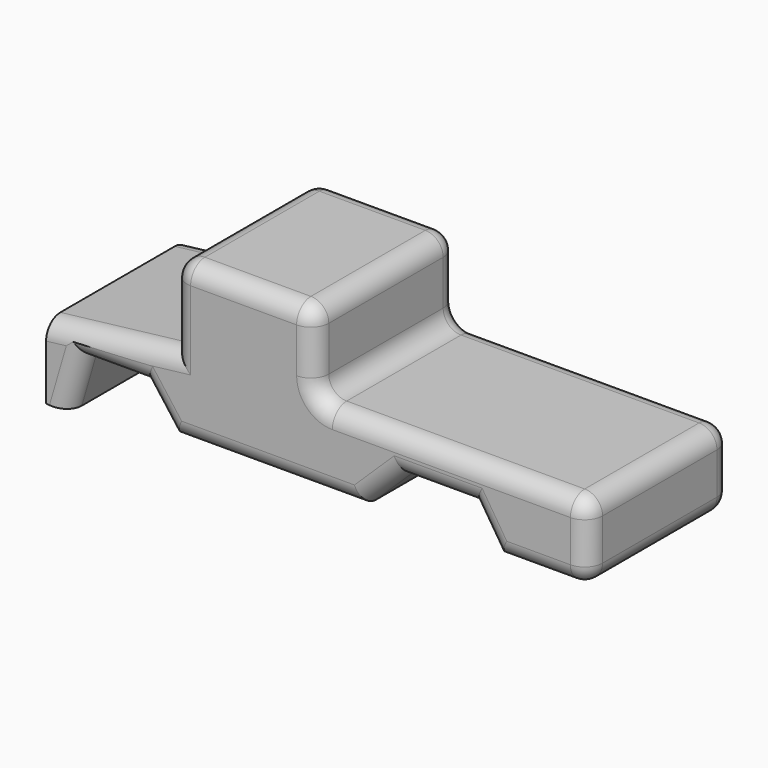
from build123d import *

# Parameters (mm, degrees)
F1_DEPTH      = 50.8
F2_T1_DEPTH   = 50.8
F2_T3_DEPTH   = 40.64
F2_T5_DEPTH   = 76.2
F2_T7_DEPTH   = 29.5973137942
F2_T9_DEPTH   = 33.5654399347
F2_T11_DEPTH  = 79.1223219872
F2_T13_DEPTH  = 47.9117414904
F2_S17_W      = 5.08
F2_S17_H      = 5.08
F2_T18_DEPTH  = 5.08
F2_S23_W      = 5.08
F2_S23_H      = 5.08
F2_T24_DEPTH  = 5.08
F2_S29_W      = 5.08
F2_S29_H      = 5.08
F2_T30_DEPTH  = 5.08
F2_S35_W      = 5.08
F2_S35_H      = 5.08
F2_T36_DEPTH  = 5.08
F2_T42_DEPTH  = 30.5130339217
F2_T47_DEPTH  = 61.6709979823
F2_T52_DEPTH  = 61.6709979823
F2_T57_DEPTH  = 30.5130339217
F2_T62_DEPTH  = 38.4398769005
F2_T67_DEPTH  = 45.5458726078
F2_T73_DEPTH  = 41.1576238629
F2_T78_DEPTH  = 38.4398769005
F2_T83_DEPTH  = 45.5458726078
F2_T89_DEPTH  = 41.1576238629
F2_T94_DEPTH  = 39.1358233333
F2_T99_DEPTH  = 42.7987075686
F2_T105_DEPTH = 40.6620223165
F2_T110_DEPTH = 39.1358233333
F2_T115_DEPTH = 42.7987075686
F2_T121_DEPTH = 40.6620223165
F2_T127_DEPTH = 30.5130339217
F2_T131_DEPTH = 61.6709979823
F2_T138_DEPTH = 30.5130339217
F2_T142_DEPTH = 61.6709979823
F2_T149_DEPTH = 38.4398769005
F2_T153_DEPTH = 45.5458726078
F2_T160_DEPTH = 41.1576238629
F2_T164_DEPTH = 45.5458726078
F2_T171_DEPTH = 38.4398769005
F2_T175_DEPTH = 45.5458726078
F2_T182_DEPTH = 41.1576238629
F2_T186_DEPTH = 45.5458726078
F2_T193_DEPTH = 42.7987075686
F2_T197_DEPTH = 39.1358233333
F2_T204_DEPTH = 40.6620223165
F2_T208_DEPTH = 42.7987075686
F2_T215_DEPTH = 42.7987075686
F2_T219_DEPTH = 39.1358233333
F2_T226_DEPTH = 40.6620223165
F2_T230_DEPTH = 42.7987075686
F2_T233_DEPTH = 12.7330339217
F2_T235_DEPTH = 67.6763198042
F2_S239_W     = 5.08
F2_S239_H     = 5.08
F2_T240_DEPTH = 5.08
F2_S245_W     = 5.08
F2_S245_H     = 5.08
F2_T246_DEPTH = 5.08
F2_S251_W     = 5.08
F2_S251_H     = 5.08
F2_T252_DEPTH = 5.08
F2_S257_W     = 5.08
F2_S257_H     = 5.08
F2_T258_DEPTH = 5.08
F2_T262_ANGLE = 90
F2_T264_ANGLE = 90


# Not quite as in the source:
# - a fillet or chamfer that OpenCascade refuses, or shapes differently, is made with other operations: its cross-section is extruded or revolved along the edge and cut away or added


with BuildPart() as f1:
    # F0 (on Front) → F1 (new body)
    with BuildSketch(Plane.XZ):
        Polygon((-106.1203256249, 11.31004747), (-106.1203256249, -9.4463042915), (-100.0155135989, -10.0567853078), (-95.7421511412, 4.5947572216), (-78.3434435725, 4.5947572216), (-70.1019465923, -6.3938992098), (-16.3796246052, -6.3938992098), (-5.0857262686, 4.5947572216), (15.0601463392, 4.5947572216), (22.0806747675, -6.3938992098), (48.0261147022, -6.3938992098), (48.0261147022, 15.5834145844), (-29.810205102, 15.5834145844), (-29.810205102, 38.4764485061), (-70.1019465923, 38.4764485061), (-70.1019465923, 15.5834145844), align=None)
    extrude(amount=F1_DEPTH)

    # F2: fillet of radius 5.08 on 33 edges, made by hand

    # F2_s2 → F2_t1 (join)
    with BuildSketch(Plane.XZ):
        with BuildLine():
            ThreePointArc((-24.730205102, 15.5834145844), (-28.3223075504, 17.071312136), (-29.810205102, 20.6634145844))
            Line((-29.810205102, 20.6634145844), (-29.810205102, 15.5834145844))
            Line((-29.810205102, 15.5834145844), (-24.730205102, 15.5834145844))
        make_face()
    extrude(amount=F2_T1_DEPTH)

    # F2_s4 → F2_t3 (cut)
    with BuildSketch(Plane.XZ.offset(5.08)):
        with BuildLine():
            ThreePointArc((-65.0219465923, 38.4764485061), (-68.6140490408, 36.9885509545), (-70.1019465923, 33.3964485061))
            Line((-70.1019465923, 33.3964485061), (-70.1019465923, 38.4764485061))
            Line((-70.1019465923, 38.4764485061), (-65.0219465923, 38.4764485061))
        make_face()
        with BuildLine():
            ThreePointArc((42.9461147022, -6.3938992098), (46.5382171507, -4.9060016582), (48.0261147022, -1.3138992098))
            Line((48.0261147022, -1.3138992098), (48.0261147022, -6.3938992098))
            Line((48.0261147022, -6.3938992098), (42.9461147022, -6.3938992098))
        make_face()
    extrude(amount=F2_T3_DEPTH, mode=Mode.SUBTRACT)

    # F2_s6 → F2_t5 (cut)
    with BuildSketch(Plane.XZ.offset(-12.7)):
        with BuildLine():
            ThreePointArc((-29.810205102, 33.3964485061), (-31.2981026535, 36.9885509545), (-34.890205102, 38.4764485061))
            Line((-34.890205102, 38.4764485061), (-29.810205102, 38.4764485061))
            Line((-29.810205102, 38.4764485061), (-29.810205102, 33.3964485061))
        make_face()
        with BuildLine():
            ThreePointArc((48.0261147022, 10.5034145844), (46.5382171507, 14.0955170328), (42.9461147022, 15.5834145844))
            Line((42.9461147022, 15.5834145844), (48.0261147022, 15.5834145844))
            Line((48.0261147022, 15.5834145844), (48.0261147022, 10.5034145844))
        make_face()
    extrude(amount=F2_T5_DEPTH, mode=Mode.SUBTRACT)

    # F2_s8 → F2_t7 (cut)
    with BuildSketch(Plane.XY.offset(-1.3138992098)):
        with BuildLine():
            ThreePointArc((48.0261147022, -5.08), (46.5382171507, -1.4878975516), (42.9461147022, 0))
            Line((42.9461147022, 0), (48.0261147022, 0))
            Line((48.0261147022, 0), (48.0261147022, -5.08))
        make_face()
        with BuildLine():
            ThreePointArc((48.0261147022, -45.72), (46.5382171507, -49.3121024484), (42.9461147022, -50.8))
            Line((42.9461147022, -50.8), (48.0261147022, -50.8))
            Line((48.0261147022, -50.8), (48.0261147022, -45.72))
        make_face()
    extrude(amount=F2_T7_DEPTH, mode=Mode.SUBTRACT)

    # F2_s10 → F2_t9 (cut)
    with BuildSketch(Plane.YZ.offset(9.3806747675)):
        with BuildLine():
            ThreePointArc((-45.72, -6.3938992098), (-49.3121024484, -4.9060016582), (-50.8, -1.3138992098))
            Line((-50.8, -1.3138992098), (-50.8, -6.3938992098))
            Line((-50.8, -6.3938992098), (-45.72, -6.3938992098))
        make_face()
        with BuildLine():
            ThreePointArc((-5.08, -6.3938992098), (-1.4878975516, -4.9060016582), (0, -1.3138992098))
            Line((0, -1.3138992098), (0, -6.3938992098))
            Line((0, -6.3938992098), (-5.08, -6.3938992098))
        make_face()
    extrude(amount=F2_T9_DEPTH, mode=Mode.SUBTRACT)

    # F2_s12 → F2_t11 (cut)
    with BuildSketch(Plane.YZ.offset(-82.8019465923)):
        with BuildLine():
            ThreePointArc((-50.8, -1.3138992098), (-49.3121024484, -4.9060016582), (-45.72, -6.3938992098))
            Line((-45.72, -6.3938992098), (-50.8, -6.3938992098))
            Line((-50.8, -6.3938992098), (-50.8, -1.3138992098))
        make_face()
        with BuildLine():
            ThreePointArc((0, -1.3138992098), (-1.4878975516, -4.9060016582), (-5.08, -6.3938992098))
            Line((-5.08, -6.3938992098), (0, -6.3938992098))
            Line((0, -6.3938992098), (0, -1.3138992098))
        make_face()
    extrude(amount=F2_T11_DEPTH, mode=Mode.SUBTRACT)

    # F2_s14 → F2_t13 (cut)
    with BuildSketch(Plane.YZ.offset(-65.0219465923)):
        with BuildLine():
            ThreePointArc((0, 33.3964485061), (-1.4878975516, 36.9885509545), (-5.08, 38.4764485061))
            Line((-5.08, 38.4764485061), (0, 38.4764485061))
            Line((0, 38.4764485061), (0, 33.3964485061))
        make_face()
        with BuildLine():
            ThreePointArc((-50.8, 33.3964485061), (-49.3121024484, 36.9885509545), (-45.72, 38.4764485061))
            Line((-45.72, 38.4764485061), (-50.8, 38.4764485061))
            Line((-50.8, 38.4764485061), (-50.8, 33.3964485061))
        make_face()
    extrude(amount=F2_T13_DEPTH, mode=Mode.SUBTRACT)


with BuildPart() as f2_tool16:
    # F2_s17 → F2_t18 (new body)
    with BuildSketch(Plane.XY.offset(33.3964485061)):
        with Locations((-67.5619465923, -2.54)):
            Rectangle(F2_S17_W, F2_S17_H)
    extrude(amount=F2_T18_DEPTH)

    # F2_s19 → F2_t20 (revolve, cut)
    with BuildSketch(Plane(origin=(-65.0219465923, -5.08, 33.3964485061), x_dir=(0.7071067812, -0.7071067812, 0), z_dir=(-0.7071067812, -0.7071067812, 0))):
        with BuildLine():
            ThreePointArc((0, -5.08), (5.08, 0), (0, 5.08))
            Line((0, 5.08), (0, -5.08))
        make_face()
    revolve(axis=Axis((-65.0219465923, -5.08, 33.3964485061), (0, 0, 1)), mode=Mode.SUBTRACT)


with BuildPart() as f1_1:
    add(f1.part)

    # F2_t15: cut F2_tool16
    add(f2_tool16.part, mode=Mode.SUBTRACT)


with BuildPart() as f2_tool22:
    # F2_s23 → F2_t24 (new body)
    with BuildSketch(Plane.XY.offset(33.3964485061)):
        with Locations((-67.5619465923, -48.26)):
            Rectangle(F2_S23_W, F2_S23_H)
    extrude(amount=F2_T24_DEPTH)

    # F2_s25 → F2_t26 (revolve, cut)
    with BuildSketch(Plane(origin=(-65.0219465923, -45.72, 33.3964485061), x_dir=(0.7071067812, 0.7071067812, 0), z_dir=(0.7071067812, -0.7071067812, 0))):
        with BuildLine():
            ThreePointArc((0, -5.08), (5.08, 0), (0, 5.08))
            Line((0, 5.08), (0, -5.08))
        make_face()
    revolve(axis=Axis((-65.0219465923, -45.72, 33.3964485061), (0, 0, 1)), mode=Mode.SUBTRACT)


with BuildPart() as f1_2:
    add(f1_1.part)

    # F2_t21: cut F2_tool22
    add(f2_tool22.part, mode=Mode.SUBTRACT)


with BuildPart() as f2_tool28:
    # F2_s29 → F2_t30 (new body)
    with BuildSketch(Plane.XY.offset(-1.3138992098)):
        with Locations((45.4861147022, -2.54)):
            Rectangle(F2_S29_W, F2_S29_H)
    extrude(amount=-F2_T30_DEPTH)

    # F2_s31 → F2_t32 (revolve, cut)
    with BuildSketch(Plane(origin=(42.9461147022, -5.08, -1.3138992098), x_dir=(-0.7071067812, -0.7071067812, 0), z_dir=(0.7071067812, -0.7071067812, 0))):
        with BuildLine():
            ThreePointArc((0, -5.08), (5.08, 0), (0, 5.08))
            Line((0, 5.08), (0, -5.08))
        make_face()
    revolve(axis=Axis((42.9461147022, -5.08, -1.3138992098), (0, 0, -1)), mode=Mode.SUBTRACT)


with BuildPart() as f1_3:
    add(f1_2.part)

    # F2_t27: cut F2_tool28
    add(f2_tool28.part, mode=Mode.SUBTRACT)


with BuildPart() as f2_tool34:
    # F2_s35 → F2_t36 (new body)
    with BuildSketch(Plane.XY.offset(-1.3138992098)):
        with Locations((45.4861147022, -48.26)):
            Rectangle(F2_S35_W, F2_S35_H)
    extrude(amount=-F2_T36_DEPTH)

    # F2_s37 → F2_t38 (revolve, cut)
    with BuildSketch(Plane(origin=(42.9461147022, -45.72, -1.3138992098), x_dir=(-0.7071067812, 0.7071067812, 0), z_dir=(-0.7071067812, -0.7071067812, 0))):
        with BuildLine():
            ThreePointArc((0, -5.08), (5.08, 0), (0, 5.08))
            Line((0, 5.08), (0, -5.08))
        make_face()
    revolve(axis=Axis((42.9461147022, -45.72, -1.3138992098), (0, 0, -1)), mode=Mode.SUBTRACT)


with BuildPart() as f1_4:
    add(f1_3.part)

    # F2_t33: cut F2_tool34
    add(f2_tool34.part, mode=Mode.SUBTRACT)


with BuildPart() as f2_tool40:
    # F2_s41 → F2_t42 (new body)
    with BuildSketch(Plane.XY.offset(33.3964485061)):
        with BuildLine():
            ThreePointArc((-65.0219465923, 0), (-68.6140490408, -1.4878975516), (-70.1019465923, -5.08))
            Line((-70.1019465923, -5.08), (-70.1019465923, 0))
            Line((-70.1019465923, 0), (-65.0219465923, 0))
        make_face()
    extrude(amount=-F2_T42_DEPTH)

    split(bisect_by=Plane(origin=(-2.796301967, 0, 23.5688302549), x_dir=(0, 1, 0), z_dir=(-0.1178177429, 0, 0.9930352358)), keep=Keep.TOP)


with BuildPart() as f1_5:
    add(f1_4.part)

    # F2_t39: cut F2_tool40
    add(f2_tool40.part, mode=Mode.SUBTRACT)


with BuildPart() as f2_tool45:
    # F2_s46 → F2_t47 (new body)
    with BuildSketch(Plane(origin=(-54.6940971312, 0, -6.4891303359), x_dir=(0, 1, 0), z_dir=(-0.9930352358, 0, -0.1178177429))):
        with BuildLine():
            ThreePointArc((0, -18.6541328949), (-1.4878975516, -22.2462353434), (-5.08, -23.7341328949))
            Line((-5.08, -23.7341328949), (0, -23.7341328949))
            Line((0, -23.7341328949), (0, -18.6541328949))
        make_face()
    extrude(amount=F2_T47_DEPTH)

    split(bisect_by=Plane.YZ.offset(-70.1019465923), keep=Keep.BOTTOM)


with BuildPart() as f1_6:
    add(f1_5.part)

    # F2_t44: cut F2_tool45
    add(f2_tool45.part, mode=Mode.SUBTRACT)


with BuildPart() as f2_tool50:
    # F2_s51 → F2_t52 (new body)
    with BuildSketch(Plane(origin=(-54.6940971312, 0, -6.4891303359), x_dir=(0, 1, 0), z_dir=(-0.9930352358, 0, -0.1178177429))):
        with BuildLine():
            ThreePointArc((-50.8, -18.6541328949), (-49.3121024484, -22.2462353434), (-45.72, -23.7341328949))
            Line((-45.72, -23.7341328949), (-50.8, -23.7341328949))
            Line((-50.8, -23.7341328949), (-50.8, -18.6541328949))
        make_face()
    extrude(amount=F2_T52_DEPTH)

    split(bisect_by=Plane.YZ.offset(-70.1019465923), keep=Keep.BOTTOM)


with BuildPart() as f1_7:
    add(f1_6.part)

    # F2_t49: cut F2_tool50
    add(f2_tool50.part, mode=Mode.SUBTRACT)


with BuildPart() as f2_tool55:
    # F2_s56 → F2_t57 (new body)
    with BuildSketch(Plane.XY.offset(33.3964485061)):
        with BuildLine():
            ThreePointArc((-65.0219465923, -50.8), (-68.6140490408, -49.3121024484), (-70.1019465923, -45.72))
            Line((-70.1019465923, -45.72), (-70.1019465923, -50.8))
            Line((-70.1019465923, -50.8), (-65.0219465923, -50.8))
        make_face()
    extrude(amount=-F2_T57_DEPTH)

    split(bisect_by=Plane(origin=(-2.796301967, 0, 23.5688302549), x_dir=(0, 1, 0), z_dir=(-0.1178177429, 0, 0.9930352358)), keep=Keep.TOP)


with BuildPart() as f1_8:
    add(f1_7.part)

    # F2_t54: cut F2_tool55
    add(f2_tool55.part, mode=Mode.SUBTRACT)


with BuildPart() as f2_tool60:
    # F2_s61 → F2_t62 (new body)
    with BuildSketch(Plane(origin=(-4.5567996099, 0, 7.1323841007), x_dir=(0, 1, 0), z_dir=(0.5383891644, 0, -0.8426963318))):
        with BuildLine():
            ThreePointArc((-45.72, 15.1648975779), (-49.3121024484, 16.6527951295), (-50.8, 20.2448975779))
            Line((-50.8, 20.2448975779), (-50.8, 15.1648975779))
            Line((-50.8, 15.1648975779), (-45.72, 15.1648975779))
        make_face()
    extrude(amount=F2_T62_DEPTH)

    split(bisect_by=Plane.XY.offset(4.5947572216), keep=Keep.BOTTOM)


with BuildPart() as f1_9:
    add(f1_8.part)

    # F2_t59: cut F2_tool60
    add(f2_tool60.part, mode=Mode.SUBTRACT)


with BuildPart() as f2_tool65:
    # F2_s66 → F2_t67 (new body)
    with BuildSketch(Plane.YZ.offset(-17.7857262686)):
        with BuildLine():
            ThreePointArc((-50.8, 9.6747572216), (-49.3121024484, 6.0826547732), (-45.72, 4.5947572216))
            Line((-45.72, 4.5947572216), (-50.8, 4.5947572216))
            Line((-50.8, 4.5947572216), (-50.8, 9.6747572216))
        make_face()
    extrude(amount=F2_T67_DEPTH)

    split(bisect_by=Plane(origin=(12.7794035613, 0, 8.1646165351), x_dir=(0, 1, 0), z_dir=(-0.8426963318, 0, -0.5383891644)), keep=Keep.TOP)

    split(bisect_by=Plane(origin=(-4.769724943, 0, 4.9022179314), x_dir=(0, 1, 0), z_dir=(0.6973549139, 0, -0.7167259756)), keep=Keep.TOP)


with BuildPart() as f1_10:
    add(f1_9.part)

    # F2_t64: cut F2_tool65
    add(f2_tool65.part, mode=Mode.SUBTRACT)


with BuildPart() as f2_tool71:
    # F2_s72 → F2_t73 (new body)
    with BuildSketch(Plane(origin=(-20.7123195525, 0, -20.1525245471), x_dir=(0, 1, 0), z_dir=(0.7167259756, 0, 0.6973549139))):
        with BuildLine():
            ThreePointArc((-50.8, 11.9197380563), (-49.3121024484, 8.3276356079), (-45.72, 6.8397380563))
            Line((-45.72, 6.8397380563), (-50.8, 6.8397380563))
            Line((-50.8, 6.8397380563), (-50.8, 11.9197380563))
        make_face()
    extrude(amount=F2_T73_DEPTH)

    split(bisect_by=Plane.XY.offset(4.5947572216), keep=Keep.BOTTOM)


with BuildPart() as f1_11:
    add(f1_10.part)

    # F2_t70: cut F2_tool71
    add(f2_tool71.part, mode=Mode.SUBTRACT)


with BuildPart() as f2_tool76:
    # F2_s77 → F2_t78 (new body)
    with BuildSketch(Plane(origin=(-4.5567996099, 0, 7.1323841007), x_dir=(0, 1, 0), z_dir=(0.5383891644, 0, -0.8426963318))):
        with BuildLine():
            ThreePointArc((-5.08, 15.1648975779), (-1.4878975516, 16.6527951295), (0, 20.2448975779))
            Line((0, 20.2448975779), (0, 15.1648975779))
            Line((0, 15.1648975779), (-5.08, 15.1648975779))
        make_face()
    extrude(amount=F2_T78_DEPTH)

    split(bisect_by=Plane.XY.offset(4.5947572216), keep=Keep.BOTTOM)


with BuildPart() as f1_12:
    add(f1_11.part)

    # F2_t75: cut F2_tool76
    add(f2_tool76.part, mode=Mode.SUBTRACT)


with BuildPart() as f2_tool81:
    # F2_s82 → F2_t83 (new body)
    with BuildSketch(Plane.YZ.offset(-17.7857262686)):
        with BuildLine():
            ThreePointArc((0, 9.6747572216), (-1.4878975516, 6.0826547732), (-5.08, 4.5947572216))
            Line((-5.08, 4.5947572216), (0, 4.5947572216))
            Line((0, 4.5947572216), (0, 9.6747572216))
        make_face()
    extrude(amount=F2_T83_DEPTH)

    split(bisect_by=Plane(origin=(12.7794035613, 0, 8.1646165351), x_dir=(0, 1, 0), z_dir=(-0.8426963318, 0, -0.5383891644)), keep=Keep.TOP)

    split(bisect_by=Plane(origin=(-4.769724943, 0, 4.9022179314), x_dir=(0, 1, 0), z_dir=(0.6973549139, 0, -0.7167259756)), keep=Keep.TOP)


with BuildPart() as f1_13:
    add(f1_12.part)

    # F2_t80: cut F2_tool81
    add(f2_tool81.part, mode=Mode.SUBTRACT)


with BuildPart() as f2_tool87:
    # F2_s88 → F2_t89 (new body)
    with BuildSketch(Plane(origin=(-20.7123195525, 0, -20.1525245471), x_dir=(0, 1, 0), z_dir=(0.7167259756, 0, 0.6973549139))):
        with BuildLine():
            ThreePointArc((0, 11.9197380563), (-1.4878975516, 8.3276356079), (-5.08, 6.8397380563))
            Line((-5.08, 6.8397380563), (0, 6.8397380563))
            Line((0, 6.8397380563), (0, 11.9197380563))
        make_face()
    extrude(amount=F2_T89_DEPTH)

    split(bisect_by=Plane.XY.offset(4.5947572216), keep=Keep.BOTTOM)


with BuildPart() as f1_14:
    add(f1_13.part)

    # F2_t86: cut F2_tool87
    add(f2_tool87.part, mode=Mode.SUBTRACT)


with BuildPart() as f2_tool92:
    # F2_s93 → F2_t94 (new body)
    with BuildSketch(Plane(origin=(-38.0291466545, 0, 50.705500223), x_dir=(0, 1, 0), z_dir=(0.600000217, 0, -0.7999998373))):
        with BuildLine():
            ThreePointArc((-50.8, -54.8378867796), (-49.3121024484, -58.429989228), (-45.72, -59.9178867796))
            Line((-45.72, -59.9178867796), (-50.8, -59.9178867796))
            Line((-50.8, -59.9178867796), (-50.8, -54.8378867796))
        make_face()
    extrude(amount=F2_T94_DEPTH)

    split(bisect_by=Plane.XY.offset(4.5947572216), keep=Keep.BOTTOM)


with BuildPart() as f1_15:
    add(f1_14.part)

    # F2_t91: cut F2_tool92
    add(f2_tool92.part, mode=Mode.SUBTRACT)


with BuildPart() as f2_tool97:
    # F2_s98 → F2_t99 (new body)
    with BuildSketch(Plane.YZ.offset(-108.4421511412)):
        with BuildLine():
            ThreePointArc((-50.8, 9.6747572216), (-49.3121024484, 6.0826547732), (-45.72, 4.5947572216))
            Line((-45.72, 4.5947572216), (-50.8, 4.5947572216))
            Line((-50.8, 4.5947572216), (-50.8, 9.6747572216))
        make_face()
    extrude(amount=F2_T99_DEPTH)

    split(bisect_by=Plane(origin=(-89.4710495478, 0, 26.0956976663), x_dir=(0, 1, 0), z_dir=(0.9600000724, 0, -0.2799997516)), keep=Keep.TOP)

    split(bisect_by=Plane(origin=(-47.9342996735, 0, -35.950745068), x_dir=(0, 1, 0), z_dir=(-0.7999998373, 0, -0.600000217)), keep=Keep.TOP)


with BuildPart() as f1_16:
    add(f1_15.part)

    # F2_t96: cut F2_tool97
    add(f2_tool97.part, mode=Mode.SUBTRACT)


with BuildPart() as f2_tool103:
    # F2_s104 → F2_t105 (new body)
    with BuildSketch(Plane(origin=(-14.1004608967, 0, -48.3444838941), x_dir=(0, 1, 0), z_dir=(0.2799997516, 0, 0.9600000724))):
        with BuildLine():
            ThreePointArc((-50.8, 98.2790029124), (-49.3121024484, 94.686900464), (-45.72, 93.1990029124))
            Line((-45.72, 93.1990029124), (-50.8, 93.1990029124))
            Line((-50.8, 93.1990029124), (-50.8, 98.2790029124))
        make_face()
    extrude(amount=F2_T105_DEPTH)

    split(bisect_by=Plane.XY.offset(4.5947572216), keep=Keep.BOTTOM)


with BuildPart() as f1_17:
    add(f1_16.part)

    # F2_t102: cut F2_tool103
    add(f2_tool103.part, mode=Mode.SUBTRACT)


with BuildPart() as f2_tool108:
    # F2_s109 → F2_t110 (new body)
    with BuildSketch(Plane(origin=(-38.0291466545, 0, 50.705500223), x_dir=(0, 1, 0), z_dir=(0.600000217, 0, -0.7999998373))):
        with BuildLine():
            ThreePointArc((0, -54.8378867796), (-1.4878975516, -58.429989228), (-5.08, -59.9178867796))
            Line((-5.08, -59.9178867796), (0, -59.9178867796))
            Line((0, -59.9178867796), (0, -54.8378867796))
        make_face()
    extrude(amount=F2_T110_DEPTH)

    split(bisect_by=Plane.XY.offset(4.5947572216), keep=Keep.BOTTOM)


with BuildPart() as f1_18:
    add(f1_17.part)

    # F2_t107: cut F2_tool108
    add(f2_tool108.part, mode=Mode.SUBTRACT)


with BuildPart() as f2_tool113:
    # F2_s114 → F2_t115 (new body)
    with BuildSketch(Plane.YZ.offset(-108.4421511412)):
        with BuildLine():
            ThreePointArc((0, 9.6747572216), (-1.4878975516, 6.0826547732), (-5.08, 4.5947572216))
            Line((-5.08, 4.5947572216), (0, 4.5947572216))
            Line((0, 4.5947572216), (0, 9.6747572216))
        make_face()
    extrude(amount=F2_T115_DEPTH)

    split(bisect_by=Plane(origin=(-89.4710495478, 0, 26.0956976663), x_dir=(0, 1, 0), z_dir=(0.9600000724, 0, -0.2799997516)), keep=Keep.TOP)

    split(bisect_by=Plane(origin=(-47.9342996735, 0, -35.950745068), x_dir=(0, 1, 0), z_dir=(-0.7999998373, 0, -0.600000217)), keep=Keep.TOP)


with BuildPart() as f1_19:
    add(f1_18.part)

    # F2_t112: cut F2_tool113
    add(f2_tool113.part, mode=Mode.SUBTRACT)


with BuildPart() as f2_tool119:
    # F2_s120 → F2_t121 (new body)
    with BuildSketch(Plane(origin=(-14.1004608967, 0, -48.3444838941), x_dir=(0, 1, 0), z_dir=(0.2799997516, 0, 0.9600000724))):
        with BuildLine():
            ThreePointArc((0, 98.2790029124), (-1.4878975516, 94.686900464), (-5.08, 93.1990029124))
            Line((-5.08, 93.1990029124), (0, 93.1990029124))
            Line((0, 93.1990029124), (0, 98.2790029124))
        make_face()
    extrude(amount=F2_T121_DEPTH)

    split(bisect_by=Plane.XY.offset(4.5947572216), keep=Keep.BOTTOM)


with BuildPart() as f1_20:
    add(f1_19.part)

    # F2_t118: cut F2_tool119
    add(f2_tool119.part, mode=Mode.SUBTRACT)


with BuildPart() as f2_tool125:
    # F2_s126 → F2_t127 (new body)
    with BuildSketch(Plane.XY.offset(33.3964485061)):
        with BuildLine():
            ThreePointArc((-65.0219465923, 0), (-68.6140490408, -1.4878975516), (-70.1019465923, -5.08))
            Line((-70.1019465923, -5.08), (-70.1019465923, 0))
            Line((-70.1019465923, 0), (-65.0219465923, 0))
        make_face()
    extrude(amount=-F2_T127_DEPTH)

    split(bisect_by=Plane(origin=(-2.796301967, 0, 23.5688302549), x_dir=(0, 1, 0), z_dir=(0.1178177429, 0, -0.9930352358)), keep=Keep.TOP)


with BuildPart() as f2_tool129:
    # F2_s130 → F2_t131 (new body)
    with BuildSketch(Plane(origin=(-54.6940971312, 0, -6.4891303359), x_dir=(0, 1, 0), z_dir=(-0.9930352358, 0, -0.1178177429))):
        with BuildLine():
            ThreePointArc((0, -18.6541328949), (-1.4878975516, -22.2462353434), (-5.08, -23.7341328949))
            Line((-5.08, -23.7341328949), (0, -23.7341328949))
            Line((0, -23.7341328949), (0, -18.6541328949))
        make_face()
    extrude(amount=F2_T131_DEPTH)

    split(bisect_by=Plane.YZ.offset(-70.1019465923), keep=Keep.TOP)


with BuildPart() as f2_tool125_1:
    add(f2_tool125.part)

    # F2_t133: intersect F2_tool129
    add(f2_tool129.part, mode=Mode.INTERSECT)


with BuildPart() as f1_21:
    add(f1_20.part)

    # F2_t123: cut F2_tool125
    add(f2_tool125_1.part, mode=Mode.SUBTRACT)


with BuildPart() as f2_tool136:
    # F2_s137 → F2_t138 (new body)
    with BuildSketch(Plane.XY.offset(33.3964485061)):
        with BuildLine():
            ThreePointArc((-65.0219465923, -50.8), (-68.6140490408, -49.3121024484), (-70.1019465923, -45.72))
            Line((-70.1019465923, -45.72), (-70.1019465923, -50.8))
            Line((-70.1019465923, -50.8), (-65.0219465923, -50.8))
        make_face()
    extrude(amount=-F2_T138_DEPTH)

    split(bisect_by=Plane(origin=(-2.796301967, 0, 23.5688302549), x_dir=(0, 1, 0), z_dir=(0.1178177429, 0, -0.9930352358)), keep=Keep.TOP)


with BuildPart() as f2_tool140:
    # F2_s141 → F2_t142 (new body)
    with BuildSketch(Plane(origin=(-54.6940971312, 0, -6.4891303359), x_dir=(0, 1, 0), z_dir=(-0.9930352358, 0, -0.1178177429))):
        with BuildLine():
            ThreePointArc((-50.8, -18.6541328949), (-49.3121024484, -22.2462353434), (-45.72, -23.7341328949))
            Line((-45.72, -23.7341328949), (-50.8, -23.7341328949))
            Line((-50.8, -23.7341328949), (-50.8, -18.6541328949))
        make_face()
    extrude(amount=F2_T142_DEPTH)

    split(bisect_by=Plane.YZ.offset(-70.1019465923), keep=Keep.TOP)


with BuildPart() as f2_tool136_1:
    add(f2_tool136.part)

    # F2_t144: intersect F2_tool140
    add(f2_tool140.part, mode=Mode.INTERSECT)


with BuildPart() as f1_22:
    add(f1_21.part)

    # F2_t134: cut F2_tool136
    add(f2_tool136_1.part, mode=Mode.SUBTRACT)


with BuildPart() as f2_tool147:
    # F2_s148 → F2_t149 (new body)
    with BuildSketch(Plane(origin=(-4.5567996099, 0, 7.1323841007), x_dir=(0, 1, 0), z_dir=(0.5383891644, 0, -0.8426963318))):
        with BuildLine():
            ThreePointArc((-45.72, 15.1648975779), (-49.3121024484, 16.6527951295), (-50.8, 20.2448975779))
            Line((-50.8, 20.2448975779), (-50.8, 15.1648975779))
            Line((-50.8, 15.1648975779), (-45.72, 15.1648975779))
        make_face()
    extrude(amount=F2_T149_DEPTH)

    split(bisect_by=Plane.XY.offset(4.5947572216), keep=Keep.TOP)


with BuildPart() as f2_tool151:
    # F2_s152 → F2_t153 (new body)
    with BuildSketch(Plane.YZ.offset(-17.7857262686)):
        with BuildLine():
            ThreePointArc((-50.8, 9.6747572216), (-49.3121024484, 6.0826547732), (-45.72, 4.5947572216))
            Line((-45.72, 4.5947572216), (-50.8, 4.5947572216))
            Line((-50.8, 4.5947572216), (-50.8, 9.6747572216))
        make_face()
    extrude(amount=F2_T153_DEPTH)

    split(bisect_by=Plane(origin=(12.7794035613, 0, 8.1646165351), x_dir=(0, 1, 0), z_dir=(0.8426963318, 0, 0.5383891644)), keep=Keep.TOP)


with BuildPart() as f2_tool147_1:
    add(f2_tool147.part)

    # F2_t155: intersect F2_tool151
    add(f2_tool151.part, mode=Mode.INTERSECT)


with BuildPart() as f1_23:
    add(f1_22.part)

    # F2_t145: cut F2_tool147
    add(f2_tool147_1.part, mode=Mode.SUBTRACT)


with BuildPart() as f2_tool158:
    # F2_s159 → F2_t160 (new body)
    with BuildSketch(Plane(origin=(-20.7123195525, 0, -20.1525245471), x_dir=(0, 1, 0), z_dir=(0.7167259756, 0, 0.6973549139))):
        with BuildLine():
            ThreePointArc((-50.8, 11.9197380563), (-49.3121024484, 8.3276356079), (-45.72, 6.8397380563))
            Line((-45.72, 6.8397380563), (-50.8, 6.8397380563))
            Line((-50.8, 6.8397380563), (-50.8, 11.9197380563))
        make_face()
    extrude(amount=F2_T160_DEPTH)

    split(bisect_by=Plane.XY.offset(4.5947572216), keep=Keep.TOP)


with BuildPart() as f2_tool162:
    # F2_s163 → F2_t164 (new body)
    with BuildSketch(Plane.YZ.offset(-17.7857262686)):
        with BuildLine():
            ThreePointArc((-50.8, 9.6747572216), (-49.3121024484, 6.0826547732), (-45.72, 4.5947572216))
            Line((-45.72, 4.5947572216), (-50.8, 4.5947572216))
            Line((-50.8, 4.5947572216), (-50.8, 9.6747572216))
        make_face()
    extrude(amount=F2_T164_DEPTH)

    split(bisect_by=Plane(origin=(-4.769724943, 0, 4.9022179314), x_dir=(0, 1, 0), z_dir=(-0.6973549139, 0, 0.7167259756)), keep=Keep.TOP)


with BuildPart() as f2_tool158_1:
    add(f2_tool158.part)

    # F2_t166: intersect F2_tool162
    add(f2_tool162.part, mode=Mode.INTERSECT)


with BuildPart() as f1_24:
    add(f1_23.part)

    # F2_t156: cut F2_tool158
    add(f2_tool158_1.part, mode=Mode.SUBTRACT)


with BuildPart() as f2_tool169:
    # F2_s170 → F2_t171 (new body)
    with BuildSketch(Plane(origin=(-4.5567996099, 0, 7.1323841007), x_dir=(0, 1, 0), z_dir=(0.5383891644, 0, -0.8426963318))):
        with BuildLine():
            ThreePointArc((-5.08, 15.1648975779), (-1.4878975516, 16.6527951295), (0, 20.2448975779))
            Line((0, 20.2448975779), (0, 15.1648975779))
            Line((0, 15.1648975779), (-5.08, 15.1648975779))
        make_face()
    extrude(amount=F2_T171_DEPTH)

    split(bisect_by=Plane.XY.offset(4.5947572216), keep=Keep.TOP)


with BuildPart() as f2_tool173:
    # F2_s174 → F2_t175 (new body)
    with BuildSketch(Plane.YZ.offset(-17.7857262686)):
        with BuildLine():
            ThreePointArc((0, 9.6747572216), (-1.4878975516, 6.0826547732), (-5.08, 4.5947572216))
            Line((-5.08, 4.5947572216), (0, 4.5947572216))
            Line((0, 4.5947572216), (0, 9.6747572216))
        make_face()
    extrude(amount=F2_T175_DEPTH)

    split(bisect_by=Plane(origin=(12.7794035613, 0, 8.1646165351), x_dir=(0, 1, 0), z_dir=(0.8426963318, 0, 0.5383891644)), keep=Keep.TOP)


with BuildPart() as f2_tool169_1:
    add(f2_tool169.part)

    # F2_t177: intersect F2_tool173
    add(f2_tool173.part, mode=Mode.INTERSECT)


with BuildPart() as f1_25:
    add(f1_24.part)

    # F2_t167: cut F2_tool169
    add(f2_tool169_1.part, mode=Mode.SUBTRACT)


with BuildPart() as f2_tool180:
    # F2_s181 → F2_t182 (new body)
    with BuildSketch(Plane(origin=(-20.7123195525, 0, -20.1525245471), x_dir=(0, 1, 0), z_dir=(0.7167259756, 0, 0.6973549139))):
        with BuildLine():
            ThreePointArc((0, 11.9197380563), (-1.4878975516, 8.3276356079), (-5.08, 6.8397380563))
            Line((-5.08, 6.8397380563), (0, 6.8397380563))
            Line((0, 6.8397380563), (0, 11.9197380563))
        make_face()
    extrude(amount=F2_T182_DEPTH)

    split(bisect_by=Plane.XY.offset(4.5947572216), keep=Keep.TOP)


with BuildPart() as f2_tool184:
    # F2_s185 → F2_t186 (new body)
    with BuildSketch(Plane.YZ.offset(-17.7857262686)):
        with BuildLine():
            ThreePointArc((0, 9.6747572216), (-1.4878975516, 6.0826547732), (-5.08, 4.5947572216))
            Line((-5.08, 4.5947572216), (0, 4.5947572216))
            Line((0, 4.5947572216), (0, 9.6747572216))
        make_face()
    extrude(amount=F2_T186_DEPTH)

    split(bisect_by=Plane(origin=(-4.769724943, 0, 4.9022179314), x_dir=(0, 1, 0), z_dir=(-0.6973549139, 0, 0.7167259756)), keep=Keep.TOP)


with BuildPart() as f2_tool180_1:
    add(f2_tool180.part)

    # F2_t188: intersect F2_tool184
    add(f2_tool184.part, mode=Mode.INTERSECT)


with BuildPart() as f1_26:
    add(f1_25.part)

    # F2_t178: cut F2_tool180
    add(f2_tool180_1.part, mode=Mode.SUBTRACT)


with BuildPart() as f2_tool191:
    # F2_s192 → F2_t193 (new body)
    with BuildSketch(Plane.YZ.offset(-108.4421511412)):
        with BuildLine():
            ThreePointArc((-50.8, 9.6747572216), (-49.3121024484, 6.0826547732), (-45.72, 4.5947572216))
            Line((-45.72, 4.5947572216), (-50.8, 4.5947572216))
            Line((-50.8, 4.5947572216), (-50.8, 9.6747572216))
        make_face()
    extrude(amount=F2_T193_DEPTH)

    split(bisect_by=Plane(origin=(-47.9342996735, 0, -35.950745068), x_dir=(0, 1, 0), z_dir=(0.7999998373, 0, 0.600000217)), keep=Keep.TOP)


with BuildPart() as f2_tool195:
    # F2_s196 → F2_t197 (new body)
    with BuildSketch(Plane(origin=(-38.0291466545, 0, 50.705500223), x_dir=(0, 1, 0), z_dir=(0.600000217, 0, -0.7999998373))):
        with BuildLine():
            ThreePointArc((-50.8, -54.8378867796), (-49.3121024484, -58.429989228), (-45.72, -59.9178867796))
            Line((-45.72, -59.9178867796), (-50.8, -59.9178867796))
            Line((-50.8, -59.9178867796), (-50.8, -54.8378867796))
        make_face()
    extrude(amount=F2_T197_DEPTH)

    split(bisect_by=Plane.XY.offset(4.5947572216), keep=Keep.TOP)


with BuildPart() as f2_tool191_1:
    add(f2_tool191.part)

    # F2_t199: intersect F2_tool195
    add(f2_tool195.part, mode=Mode.INTERSECT)


with BuildPart() as f1_27:
    add(f1_26.part)

    # F2_t189: cut F2_tool191
    add(f2_tool191_1.part, mode=Mode.SUBTRACT)


with BuildPart() as f2_tool202:
    # F2_s203 → F2_t204 (new body)
    with BuildSketch(Plane(origin=(-14.1004608967, 0, -48.3444838941), x_dir=(0, 1, 0), z_dir=(0.2799997516, 0, 0.9600000724))):
        with BuildLine():
            ThreePointArc((-50.8, 98.2790029124), (-49.3121024484, 94.686900464), (-45.72, 93.1990029124))
            Line((-45.72, 93.1990029124), (-50.8, 93.1990029124))
            Line((-50.8, 93.1990029124), (-50.8, 98.2790029124))
        make_face()
    extrude(amount=F2_T204_DEPTH)

    split(bisect_by=Plane.XY.offset(4.5947572216), keep=Keep.TOP)


with BuildPart() as f2_tool206:
    # F2_s207 → F2_t208 (new body)
    with BuildSketch(Plane.YZ.offset(-108.4421511412)):
        with BuildLine():
            ThreePointArc((-50.8, 9.6747572216), (-49.3121024484, 6.0826547732), (-45.72, 4.5947572216))
            Line((-45.72, 4.5947572216), (-50.8, 4.5947572216))
            Line((-50.8, 4.5947572216), (-50.8, 9.6747572216))
        make_face()
    extrude(amount=F2_T208_DEPTH)

    split(bisect_by=Plane(origin=(-89.4710495478, 0, 26.0956976663), x_dir=(0, 1, 0), z_dir=(-0.9600000724, 0, 0.2799997516)), keep=Keep.TOP)


with BuildPart() as f2_tool202_1:
    add(f2_tool202.part)

    # F2_t210: intersect F2_tool206
    add(f2_tool206.part, mode=Mode.INTERSECT)


with BuildPart() as f1_28:
    add(f1_27.part)

    # F2_t200: cut F2_tool202
    add(f2_tool202_1.part, mode=Mode.SUBTRACT)


with BuildPart() as f2_tool213:
    # F2_s214 → F2_t215 (new body)
    with BuildSketch(Plane.YZ.offset(-108.4421511412)):
        with BuildLine():
            ThreePointArc((0, 9.6747572216), (-1.4878975516, 6.0826547732), (-5.08, 4.5947572216))
            Line((-5.08, 4.5947572216), (0, 4.5947572216))
            Line((0, 4.5947572216), (0, 9.6747572216))
        make_face()
    extrude(amount=F2_T215_DEPTH)

    split(bisect_by=Plane(origin=(-47.9342996735, 0, -35.950745068), x_dir=(0, 1, 0), z_dir=(0.7999998373, 0, 0.600000217)), keep=Keep.TOP)


with BuildPart() as f2_tool217:
    # F2_s218 → F2_t219 (new body)
    with BuildSketch(Plane(origin=(-38.0291466545, 0, 50.705500223), x_dir=(0, 1, 0), z_dir=(0.600000217, 0, -0.7999998373))):
        with BuildLine():
            ThreePointArc((0, -54.8378867796), (-1.4878975516, -58.429989228), (-5.08, -59.9178867796))
            Line((-5.08, -59.9178867796), (0, -59.9178867796))
            Line((0, -59.9178867796), (0, -54.8378867796))
        make_face()
    extrude(amount=F2_T219_DEPTH)

    split(bisect_by=Plane.XY.offset(4.5947572216), keep=Keep.TOP)


with BuildPart() as f2_tool213_1:
    add(f2_tool213.part)

    # F2_t221: intersect F2_tool217
    add(f2_tool217.part, mode=Mode.INTERSECT)


with BuildPart() as f1_29:
    add(f1_28.part)

    # F2_t211: cut F2_tool213
    add(f2_tool213_1.part, mode=Mode.SUBTRACT)


with BuildPart() as f2_tool224:
    # F2_s225 → F2_t226 (new body)
    with BuildSketch(Plane(origin=(-14.1004608967, 0, -48.3444838941), x_dir=(0, 1, 0), z_dir=(0.2799997516, 0, 0.9600000724))):
        with BuildLine():
            ThreePointArc((0, 98.2790029124), (-1.4878975516, 94.686900464), (-5.08, 93.1990029124))
            Line((-5.08, 93.1990029124), (0, 93.1990029124))
            Line((0, 93.1990029124), (0, 98.2790029124))
        make_face()
    extrude(amount=F2_T226_DEPTH)

    split(bisect_by=Plane.XY.offset(4.5947572216), keep=Keep.TOP)


with BuildPart() as f2_tool228:
    # F2_s229 → F2_t230 (new body)
    with BuildSketch(Plane.YZ.offset(-108.4421511412)):
        with BuildLine():
            ThreePointArc((0, 9.6747572216), (-1.4878975516, 6.0826547732), (-5.08, 4.5947572216))
            Line((-5.08, 4.5947572216), (0, 4.5947572216))
            Line((0, 4.5947572216), (0, 9.6747572216))
        make_face()
    extrude(amount=F2_T230_DEPTH)

    split(bisect_by=Plane(origin=(-89.4710495478, 0, 26.0956976663), x_dir=(0, 1, 0), z_dir=(-0.9600000724, 0, 0.2799997516)), keep=Keep.TOP)


with BuildPart() as f2_tool224_1:
    add(f2_tool224.part)

    # F2_t232: intersect F2_tool228
    add(f2_tool228.part, mode=Mode.INTERSECT)


with BuildPart() as f1_30:
    add(f1_29.part)

    # F2_t222: cut F2_tool224
    add(f2_tool224_1.part, mode=Mode.SUBTRACT)

    # F2_s234 → F2_t233 (cut)
    with BuildSketch(Plane.XY.offset(20.6634145844)):
        with BuildLine():
            ThreePointArc((-34.890205102, -50.8), (-31.2981026535, -49.3121024484), (-29.810205102, -45.72))
            Line((-29.810205102, -45.72), (-29.810205102, -50.8))
            Line((-29.810205102, -50.8), (-34.890205102, -50.8))
        make_face()
        with BuildLine():
            ThreePointArc((-29.810205102, -5.08), (-31.2981026535, -1.4878975516), (-34.890205102, 0))
            Line((-34.890205102, 0), (-29.810205102, 0))
            Line((-29.810205102, 0), (-29.810205102, -5.08))
        make_face()
    extrude(amount=F2_T233_DEPTH, mode=Mode.SUBTRACT)

    # F2_s236 → F2_t235 (cut)
    with BuildSketch(Plane.YZ.offset(-24.730205102)):
        with BuildLine():
            ThreePointArc((0, 10.5034145844), (-1.4878975516, 14.0955170328), (-5.08, 15.5834145844))
            Line((-5.08, 15.5834145844), (0, 15.5834145844))
            Line((0, 15.5834145844), (0, 10.5034145844))
        make_face()
        with BuildLine():
            ThreePointArc((-50.8, 10.5034145844), (-49.3121024484, 14.0955170328), (-45.72, 15.5834145844))
            Line((-45.72, 15.5834145844), (-50.8, 15.5834145844))
            Line((-50.8, 15.5834145844), (-50.8, 10.5034145844))
        make_face()
    extrude(amount=F2_T235_DEPTH, mode=Mode.SUBTRACT)


with BuildPart() as f2_tool238:
    # F2_s239 → F2_t240 (new body)
    with BuildSketch(Plane.XZ.offset(45.72)):
        with Locations((45.4861147022, 13.0434145844)):
            Rectangle(F2_S239_W, F2_S239_H)
    extrude(amount=F2_T240_DEPTH)

    # F2_s241 → F2_t242 (revolve, cut)
    with BuildSketch(Plane(origin=(42.9461147022, -45.72, 10.5034145844), x_dir=(-0.7071067812, 0, -0.7071067812), z_dir=(-0.7071067812, 0, 0.7071067812))):
        with BuildLine():
            ThreePointArc((0, -5.08), (5.08, 0), (0, 5.08))
            Line((0, 5.08), (0, -5.08))
        make_face()
    revolve(axis=Axis((42.9461147022, -45.72, 10.5034145844), (0, -1, 0)), mode=Mode.SUBTRACT)


with BuildPart() as f1_31:
    add(f1_30.part)

    # F2_t237: cut F2_tool238
    add(f2_tool238.part, mode=Mode.SUBTRACT)


with BuildPart() as f2_tool244:
    # F2_s245 → F2_t246 (new body)
    with BuildSketch(Plane.XZ.offset(5.08)):
        with Locations((45.4861147022, 13.0434145844)):
            Rectangle(F2_S245_W, F2_S245_H)
    extrude(amount=-F2_T246_DEPTH)

    # F2_s247 → F2_t248 (revolve, cut)
    with BuildSketch(Plane(origin=(42.9461147022, -5.08, 10.5034145844), x_dir=(-0.7071067812, 0, -0.7071067812), z_dir=(0.7071067812, 0, -0.7071067812))):
        with BuildLine():
            ThreePointArc((0, -5.08), (5.08, 0), (0, 5.08))
            Line((0, 5.08), (0, -5.08))
        make_face()
    revolve(axis=Axis((42.9461147022, -5.08, 10.5034145844), (0, 1, 0)), mode=Mode.SUBTRACT)


with BuildPart() as f1_32:
    add(f1_31.part)

    # F2_t243: cut F2_tool244
    add(f2_tool244.part, mode=Mode.SUBTRACT)


with BuildPart() as f2_tool250:
    # F2_s251 → F2_t252 (new body)
    with BuildSketch(Plane.YZ.offset(-34.890205102)):
        with Locations((-2.54, 35.9364485061)):
            Rectangle(F2_S251_W, F2_S251_H)
    extrude(amount=F2_T252_DEPTH)

    # F2_s253 → F2_t254 (revolve, cut)
    with BuildSketch(Plane(origin=(-34.890205102, -5.08, 33.3964485061), x_dir=(0, -0.7071067812, -0.7071067812), z_dir=(0, -0.7071067812, 0.7071067812))):
        with BuildLine():
            ThreePointArc((0, -5.08), (5.08, 0), (0, 5.08))
            Line((0, 5.08), (0, -5.08))
        make_face()
    revolve(axis=Axis((-34.890205102, -5.08, 33.3964485061), (1, 0, 0)), mode=Mode.SUBTRACT)


with BuildPart() as f1_33:
    add(f1_32.part)

    # F2_t249: cut F2_tool250
    add(f2_tool250.part, mode=Mode.SUBTRACT)


with BuildPart() as f2_tool256:
    # F2_s257 → F2_t258 (new body)
    with BuildSketch(Plane.XZ.offset(45.72)):
        with Locations((-32.350205102, 35.9364485061)):
            Rectangle(F2_S257_W, F2_S257_H)
    extrude(amount=F2_T258_DEPTH)

    # F2_s259 → F2_t260 (revolve, cut)
    with BuildSketch(Plane(origin=(-34.890205102, -45.72, 33.3964485061), x_dir=(-0.7071067812, 0, -0.7071067812), z_dir=(-0.7071067812, 0, 0.7071067812))):
        with BuildLine():
            ThreePointArc((0, -5.08), (5.08, 0), (0, 5.08))
            Line((0, 5.08), (0, -5.08))
        make_face()
    revolve(axis=Axis((-34.890205102, -45.72, 33.3964485061), (0, -1, 0)), mode=Mode.SUBTRACT)


with BuildPart() as f1_34:
    add(f1_33.part)

    # F2_t255: cut F2_tool256
    add(f2_tool256.part, mode=Mode.SUBTRACT)

    # F2_s261 → F2_t262 (revolve, cut)
    with BuildSketch(Plane.YZ.offset(-24.730205102)):
        with BuildLine():
            ThreePointArc((-50.8, 10.5034145844), (-49.3121024484, 14.0955170328), (-45.72, 15.5834145844))
            Line((-45.72, 15.5834145844), (-50.8, 15.5834145844))
            Line((-50.8, 15.5834145844), (-50.8, 10.5034145844))
        make_face()
    revolve(axis=Axis((-24.730205102, -50.8, 20.6634145844), (0, 1, 0)), revolution_arc=F2_T262_ANGLE, mode=Mode.SUBTRACT)

    # F2_s263 → F2_t264 (revolve, cut)
    with BuildSketch(Plane.YZ.offset(-24.730205102)):
        with BuildLine():
            ThreePointArc((0, 10.5034145844), (-1.4878975516, 14.0955170328), (-5.08, 15.5834145844))
            Line((-5.08, 15.5834145844), (0, 15.5834145844))
            Line((0, 15.5834145844), (0, 10.5034145844))
        make_face()
    revolve(axis=Axis((-24.730205102, 0, 20.6634145844), (0, 1, 0)), revolution_arc=F2_T264_ANGLE, mode=Mode.SUBTRACT)


solid = f1_34.part
